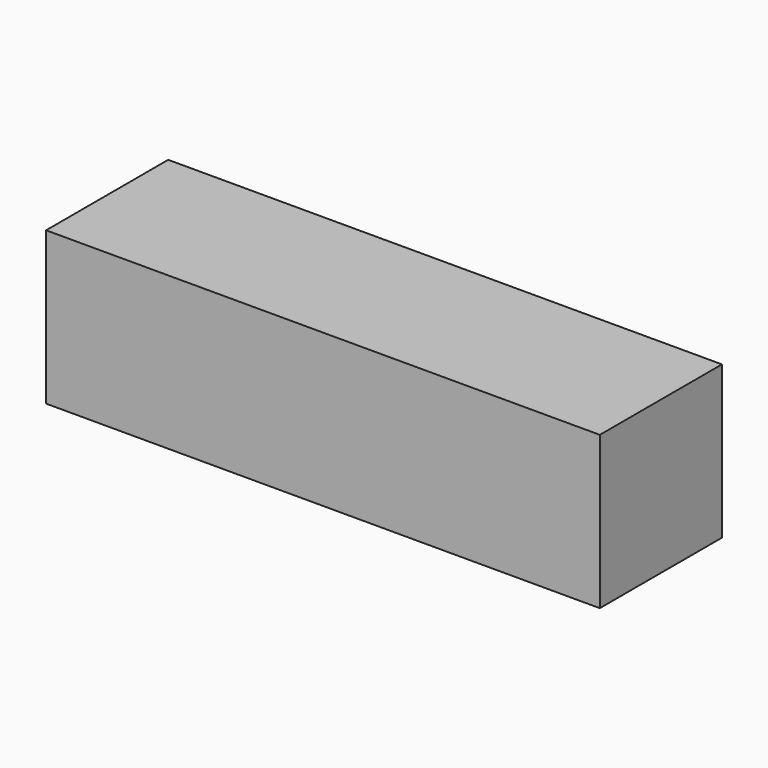
from build123d import *

# Parameters (mm, degrees)
F1_E0_BOTTOM_W = 92.1574085951
F1_E0_BOTTOM_H = 25.4
F2_DEPTH       = 25.4


with BuildPart() as f2:
    # F1_E0_bottom (on explicit) → F2 (new body)
    with BuildSketch(Plane(origin=(-40.7175570726, 0, 33.8634364307), x_dir=(1, 0, 0), z_dir=(0, 0, 1))):
        with Locations((46.0787042975, 12.7)):
            Rectangle(F1_E0_BOTTOM_W, F1_E0_BOTTOM_H)
    extrude(amount=F2_DEPTH)


solid = f2.part
